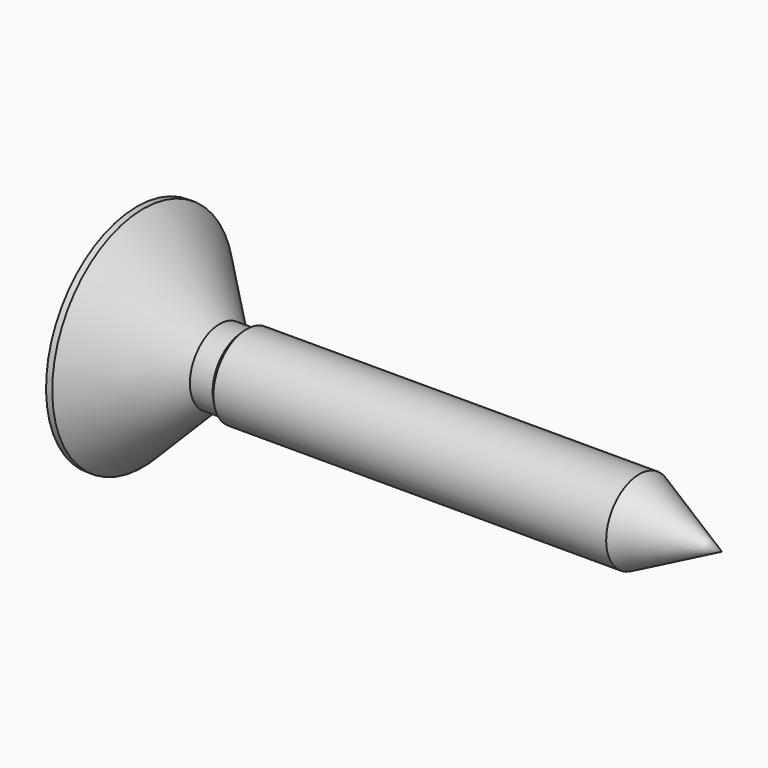
from build123d import *

# Parameters (mm, degrees)
F3_DEPTH = 0.5


# Not quite as in the source:
# - a pattern or mirror of a feature is missing from the dataset's text; its kind, count and spacing are read off the source's solid


with BuildPart() as f1:
    # F0 (on Front) → F1 (revolve)
    with BuildSketch(Plane.XZ):
        with BuildLine():
            Line((28, 0), (24, 2))
            Line((24, 2), (5, 2))
            Line((5, 2), (4.8, 1.8))
            Line((4.8, 1.8), (3.7, 1.8))
            Line((3.7, 1.8), (0, 5.5))
            Line((0, 5.5), (-0.3, 5.5))
            ThreePointArc((-0.3, 5.5), (-1.196512283, 2.814693589), (-1.5, 0))
            Line((-1.5, 0), (28, 0))
        make_face()
    revolve(axis=Axis((13.25, 0, 0), (-1, 0, 0)))

    # F2 (on Front) → F3 (cut, symmetric)
    with BuildSketch(Plane.XZ):
        Polygon((-1.2611724095, 2.5), (-1.5, 2.5), (-1.5, 0), (-1.5, -2.5), (-1.2611724095, -2.5), (1, -0.5), (1, 0), (1, 0.5), align=None)
    f3 = extrude(amount=F3_DEPTH, both=True, mode=Mode.SUBTRACT)

    # F3_copies: F3 across plane
    add(f3.mirror(Plane(origin=(0, 0, 0), x_dir=(0, 0.7071067832, 0.7071067792), z_dir=(4.5e-09, -0.7071067792, 0.7071067832))), mode=Mode.SUBTRACT)


solid = f1.part
